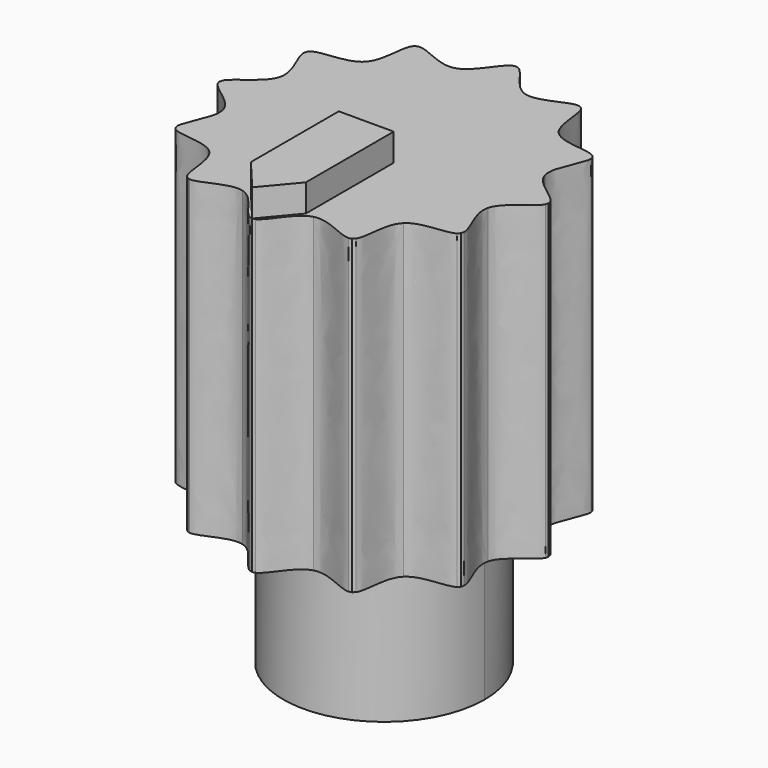
from build123d import *
from build123d import SkipClean  # not in build123d's __all__

# Parameters (mm, degrees)
F1_DEPTH = 17
F2_DEPTH = 8
F3_DEPTH = 4
F5_DEPTH = 1.5


# Not quite as in the source:
# - after a boolean that leaves OpenCascade's solid faulty, fix() repairs it
# - a feature names something its author has since deleted; it is built from what else it names


with BuildPart() as f1:
    # F0 (on Top) → F1 (new body)
    with BuildSketch(Plane.XY):
        Polygon((-7.2445266217, 1.9408333333), (-7.2443607594, -1.9414523397), (-5.303074282, -5.3035274261), (-1.9408333333, -7.2445266217), (1.9414523397, -7.2443607594), (5.3035274261, -5.303074282), (7.2445266217, -1.9408333333), (7.2443607594, 1.9414523397), (5.303074282, 5.3035274261), (1.9408333333, 7.2445266217), (-1.9414523397, 7.2443607594), (-5.3035274261, 5.303074282), align=None)
        with BuildLine():
            ThreePointArc((-3.95, 3.8272052467), (2.0645822822, 5.0977936404), (5.5, 0))
            ThreePointArc((5.5, 0), (2.0645822822, -5.0977936404), (-3.95, -3.8272052467))
            ThreePointArc((-3.95, -3.8272052467), (-5.5, 0), (-3.95, 3.8272052467))
        make_face(mode=Mode.SUBTRACT)
        with BuildLine():
            ThreePointArc((-3.95, -3.8272052467), (2.0645822822, -5.0977936404), (5.5, 0))
            ThreePointArc((5.5, 0), (2.0645822822, 5.0977936404), (-3.95, 3.8272052467))
            Line((-3.95, 3.8272052467), (-3.95, -3.8272052467))
        make_face()
        with BuildLine():
            Line((-1.85, -2.8526303651), (-1.85, 2.8526303651))
            ThreePointArc((-1.85, 2.8526303651), (3.4, 0), (-1.85, -2.8526303651))
        make_face(mode=Mode.SUBTRACT)
        with BuildLine():
            ThreePointArc((-1.85, -2.8526303651), (3.4, 0), (-1.85, 2.8526303651))
            Line((-1.85, 2.8526303651), (-1.85, -2.8526303651))
        make_face()
        with BuildLine():
            Line((-3.95, -3.8272052467), (-3.95, 3.8272052467))
            ThreePointArc((-3.95, 3.8272052467), (-5.5, 0), (-3.95, -3.8272052467))
        make_face()
        with BuildLine():
            add(Edge.make_bspline(
                [(5.303074282, 5.3035274261), (5.8806686185, 4.7260804431), (7.2203514603, 4.9114598493), (7.6765424159, 4.6182190274)],
                knots=[0.1250207704, 0.1250207704, 0.1250207704, 0.1250207704, 0.1625294045, 0.1625294045, 0.1625294045, 0.1625294045], degree=3))
            Line((5.303074282, 5.3035274261), (7.2443607594, 1.9414523397))
            add(Edge.make_bspline(
                [(7.836712211, 4.338802441), (7.8605022236, 3.7962755696), (7.0343491304, 2.7298107055), (7.2443607594, 1.9414523397)],
                knots=[0.1709157668, 0.1709157668, 0.1709157668, 0.1709157668, 0.2083694642, 0.2083694642, 0.2083694642, 0.2083694642], degree=3))
            Line((7.836712211, 4.338802441), (7.7934595092, 4.5013319004))
            Line((7.7934595092, 4.5013319004), (7.6765424159, 4.6182190274))
        make_face()
        with BuildLine():
            Line((7.2445266217, -1.9408333333), (5.3035274261, -5.303074282))
            add(Edge.make_bspline(
                [(7.6765915068, -4.6181699492), (7.2205093081, -4.9113554899), (5.8811502119, -4.725750538), (5.3035274261, -5.303074282)],
                knots=[0.3374691289, 0.3374691289, 0.3374691289, 0.3374691289, 0.3749746888, 0.3749746888, 0.3749746888, 0.3749746888], degree=3))
            Line((7.6765915068, -4.6181699492), (7.7934595092, -4.5013319004))
            Line((7.7934595092, -4.5013319004), (7.8367302299, -4.3387347317))
            add(Edge.make_bspline(
                [(7.2445266217, -1.9408333333), (7.0343944918, -2.729228444), (7.8605138313, -3.7960853183), (7.8367302299, -4.3387347317)],
                knots=[0.2916259951, 0.2916259951, 0.2916259951, 0.2916259951, 0.3290827591, 0.3290827591, 0.3290827591, 0.3290827591], degree=3))
        make_face()
        with BuildLine():
            Line((-7.836712211, -4.338802441), (-7.7934595092, -4.5013319004))
            Line((-7.7934595092, -4.5013319004), (-7.6765424159, -4.6182190274))
            add(Edge.make_bspline(
                [(-5.303074282, -5.3035274261), (-5.8806686185, -4.7260804431), (-7.2203514603, -4.9114598493), (-7.6765424159, -4.6182190274)],
                knots=[0.6250207704, 0.6250207704, 0.6250207704, 0.6250207704, 0.6625294045, 0.6625294045, 0.6625294045, 0.6625294045], degree=3))
            Line((-5.303074282, -5.3035274261), (-7.2443607594, -1.9414523397))
            add(Edge.make_bspline(
                [(-7.836712211, -4.338802441), (-7.8605022236, -3.7962755696), (-7.0343491304, -2.7298107055), (-7.2443607594, -1.9414523397)],
                knots=[0.6709157668, 0.6709157668, 0.6709157668, 0.6709157668, 0.7083694642, 0.7083694642, 0.7083694642, 0.7083694642], degree=3))
        make_face()
        with BuildLine():
            add(Edge.make_bspline(
                [(-7.2445266217, 1.9408333333), (-7.0343944918, 2.729228444), (-7.8605138313, 3.7960853183), (-7.8367302299, 4.3387347317)],
                knots=[0.7916259951, 0.7916259951, 0.7916259951, 0.7916259951, 0.8290827591, 0.8290827591, 0.8290827591, 0.8290827591], degree=3))
            Line((-7.2445266217, 1.9408333333), (-5.3035274261, 5.303074282))
            add(Edge.make_bspline(
                [(-7.6765915068, 4.6181699492), (-7.2205093081, 4.9113554899), (-5.8811502119, 4.725750538), (-5.3035274261, 5.303074282)],
                knots=[0.8374691289, 0.8374691289, 0.8374691289, 0.8374691289, 0.8749746888, 0.8749746888, 0.8749746888, 0.8749746888], degree=3))
            Line((-7.6765915068, 4.6181699492), (-7.7934595092, 4.5013319004))
            Line((-7.7934595092, 4.5013319004), (-7.8367302299, 4.3387347317))
        make_face()
        with BuildLine():
            add(Edge.make_bspline(
                [(-5.3035274261, 5.303074282), (-4.7259202525, 5.8803824219), (-4.9100082127, 7.220578017), (-4.616771189, 7.6772060222)],
                knots=[0.8749746888, 0.8749746888, 0.8749746888, 0.8749746888, 0.912479235, 0.912479235, 0.912479235, 0.912479235], degree=3))
            Line((-5.3035274261, 5.303074282), (-1.9414523397, 7.2443607594))
            add(Edge.make_bspline(
                [(-4.3392026037, 7.8375128572), (-3.7975030713, 7.8631116303), (-2.7301851448, 7.0331622426), (-1.9414523397, 7.2443607594)],
                knots=[0.9208262715, 0.9208262715, 0.9208262715, 0.9208262715, 0.9583233826, 0.9583233826, 0.9583233826, 0.9583233826], degree=3))
            Line((-4.3392026037, 7.8375128572), (-4.4993340005, 7.7946131111))
            Line((-4.4993340005, 7.7946131111), (-4.616771189, 7.6772060222))
        make_face()
        with BuildLine():
            add(Edge.make_bspline(
                [(1.9408333333, 7.2445266217), (2.7296030644, 7.0332071753), (3.7973140152, 7.8631231549), (4.3391354979, 7.8375308351)],
                knots=[0.0416720765, 0.0416720765, 0.0416720765, 0.0416720765, 0.0791722617, 0.0791722617, 0.0791722617, 0.0791722617], degree=3))
            Line((1.9408333333, 7.2445266217), (5.303074282, 5.3035274261))
            add(Edge.make_bspline(
                [(4.6167220822, 7.6772551165), (4.9099036808, 7.2207359364), (4.7255902419, 5.8808641408), (5.303074282, 5.3035274261)],
                knots=[0.087519299, 0.087519299, 0.087519299, 0.087519299, 0.1250207704, 0.1250207704, 0.1250207704, 0.1250207704], degree=3))
            Line((4.6167220822, 7.6772551165), (4.4993340005, 7.7946131111))
            Line((4.4993340005, 7.7946131111), (4.3391354979, 7.8375308351))
        make_face()
        with BuildLine():
            Line((5.3035274261, -5.303074282), (1.9414523397, -7.2443607594))
            add(Edge.make_bspline(
                [(4.3392026037, -7.8375128572), (3.7975030713, -7.8631116303), (2.7301851448, -7.0331622426), (1.9414523397, -7.2443607594)],
                knots=[0.4208262715, 0.4208262715, 0.4208262715, 0.4208262715, 0.4583233826, 0.4583233826, 0.4583233826, 0.4583233826], degree=3))
            Line((4.3392026037, -7.8375128572), (4.4993340005, -7.7946131111))
            Line((4.4993340005, -7.7946131111), (4.616771189, -7.6772060222))
            add(Edge.make_bspline(
                [(5.3035274261, -5.303074282), (4.7259202525, -5.8803824219), (4.9100082127, -7.220578017), (4.616771189, -7.6772060222)],
                knots=[0.3749746888, 0.3749746888, 0.3749746888, 0.3749746888, 0.412479235, 0.412479235, 0.412479235, 0.412479235], degree=3))
        make_face()
        with BuildLine():
            add(Edge.make_bspline(
                [(-4.6167220822, -7.6772551165), (-4.9099036808, -7.2207359364), (-4.7255902419, -5.8808641408), (-5.303074282, -5.3035274261)],
                knots=[0.587519299, 0.587519299, 0.587519299, 0.587519299, 0.6250207704, 0.6250207704, 0.6250207704, 0.6250207704], degree=3))
            Line((-4.6167220822, -7.6772551165), (-4.4993340005, -7.7946131111))
            Line((-4.4993340005, -7.7946131111), (-4.3391354979, -7.8375308351))
            add(Edge.make_bspline(
                [(-1.9408333333, -7.2445266217), (-2.7296030644, -7.0332071753), (-3.7973140152, -7.8631231549), (-4.3391354979, -7.8375308351)],
                knots=[0.5416720765, 0.5416720765, 0.5416720765, 0.5416720765, 0.5791722617, 0.5791722617, 0.5791722617, 0.5791722617], degree=3))
            Line((-1.9408333333, -7.2445266217), (-5.303074282, -5.3035274261))
        make_face()
        with BuildLine():
            add(Edge.make_bspline(
                [(-1.9414523397, 7.2443607594), (-1.1526036351, 7.4555903106), (-0.6424219306, 8.7082737692), (-0.1602865257, 8.9570586944)],
                knots=[0.9583233826, 0.9583233826, 0.9583233826, 0.9583233826, 0.9958260038, 0.9958260038, 0.9958260038, 0.9958260038], degree=3))
            Line((-1.9414523397, 7.2443607594), (1.9408333333, 7.2445266217))
            add(Edge.make_bspline(
                [(0.1602194418, 8.9570766663), (0.6422524515, 8.7083582889), (1.1520770317, 7.4558424701), (1.9408333333, 7.2445266217)],
                knots=[0.0041725298, 0.0041725298, 0.0041725298, 0.0041725298, 0.0416720765, 0.0416720765, 0.0416720765, 0.0416720765], degree=3))
            Line((0.1602194418, 8.9570766663), (0, 9))
            Line((0, 9), (-0.1602865257, 8.9570586944))
        make_face()
        with BuildLine():
            Line((1.9414523397, -7.2443607594), (-1.9408333333, -7.2445266217))
            add(Edge.make_bspline(
                [(-0.1602194418, -8.9570766663), (-0.6422524515, -8.7083582889), (-1.1520770317, -7.4558424701), (-1.9408333333, -7.2445266217)],
                knots=[0.5041725298, 0.5041725298, 0.5041725298, 0.5041725298, 0.5416720765, 0.5416720765, 0.5416720765, 0.5416720765], degree=3))
            Line((-0.1602194418, -8.9570766663), (0, -9))
            Line((0, -9), (0.1602865257, -8.9570586944))
            add(Edge.make_bspline(
                [(1.9414523397, -7.2443607594), (1.1526036351, -7.4555903106), (0.6424219306, -8.7082737692), (0.1602865257, -8.9570586944)],
                knots=[0.4583233826, 0.4583233826, 0.4583233826, 0.4583233826, 0.4958260038, 0.4958260038, 0.4958260038, 0.4958260038], degree=3))
        make_face()
        with BuildLine():
            Line((7.2443607594, 1.9414523397), (7.2445266217, -1.9408333333))
            add(Edge.make_bspline(
                [(8.9487800371, -0.160016485), (8.7015742639, -0.6422872861), (7.4547035861, -1.1522700079), (7.2445266217, -1.9408333333)],
                knots=[0.2541612392, 0.2541612392, 0.2541612392, 0.2541612392, 0.2916259951, 0.2916259951, 0.2916259951, 0.2916259951], degree=3))
            Line((8.9487800371, -0.160016485), (8.9913639805, 0))
            Line((8.9913639805, 0), (8.948762183, 0.1600835748))
            add(Edge.make_bspline(
                [(7.2443607594, 1.9414523397), (7.4544516979, 1.1527962558), (8.701490107, 0.6424567599), (8.948762183, 0.1600835748)],
                knots=[0.2083694642, 0.2083694642, 0.2083694642, 0.2083694642, 0.2458373058, 0.2458373058, 0.2458373058, 0.2458373058], degree=3))
        make_face()
        with BuildLine():
            Line((-8.9913639805, 0), (-8.948762183, -0.1600835748))
            add(Edge.make_bspline(
                [(-7.2443607594, -1.9414523397), (-7.4544516979, -1.1527962558), (-8.701490107, -0.6424567599), (-8.948762183, -0.1600835748)],
                knots=[0.7083694642, 0.7083694642, 0.7083694642, 0.7083694642, 0.7458373058, 0.7458373058, 0.7458373058, 0.7458373058], degree=3))
            Line((-7.2443607594, -1.9414523397), (-7.2445266217, 1.9408333333))
            add(Edge.make_bspline(
                [(-8.9487800371, 0.160016485), (-8.7015742639, 0.6422872861), (-7.4547035861, 1.1522700079), (-7.2445266217, 1.9408333333)],
                knots=[0.7541612392, 0.7541612392, 0.7541612392, 0.7541612392, 0.7916259951, 0.7916259951, 0.7916259951, 0.7916259951], degree=3))
            Line((-8.9487800371, 0.160016485), (-8.9913639805, 0))
        make_face()
    extrude(amount=F1_DEPTH)

    # F0 (on Top) → F2 (join)
    with BuildSketch(Plane.XY):
        with BuildLine():
            ThreePointArc((-3.95, -3.8272052467), (2.0645822822, -5.0977936404), (5.5, 0))
            ThreePointArc((5.5, 0), (2.0645822822, 5.0977936404), (-3.95, 3.8272052467))
            Line((-3.95, 3.8272052467), (-3.95, -3.8272052467))
        make_face()
        with BuildLine():
            Line((-1.85, -2.8526303651), (-1.85, 2.8526303651))
            ThreePointArc((-1.85, 2.8526303651), (3.4, 0), (-1.85, -2.8526303651))
        make_face(mode=Mode.SUBTRACT)
    extrude(amount=-F2_DEPTH)

    # F0 (on Top) → F3 (cut)
    with BuildSketch(Plane.XY):
        with BuildLine():
            ThreePointArc((-1.85, -2.8526303651), (3.4, 0), (-1.85, 2.8526303651))
            Line((-1.85, 2.8526303651), (-1.85, -2.8526303651))
        make_face()
    with SkipClean():  # cleaning this boolean's faces spoils the solid; the shape is the same uncleaned
        extrude(amount=F3_DEPTH, mode=Mode.SUBTRACT)

    # F4 (on face) → F5 (join)
    with BuildSketch(Plane.XY.offset(17)):
        Polygon((-1.5, -1.2123696111), (-1.5, -7.2123696111), (0, -9), (1.5, -7.2123696111), (1.5, -1.2123696111), align=None)
    extrude(amount=F5_DEPTH)

    add(f1.part.fix(), mode=Mode.REPLACE)


solid = f1.part
